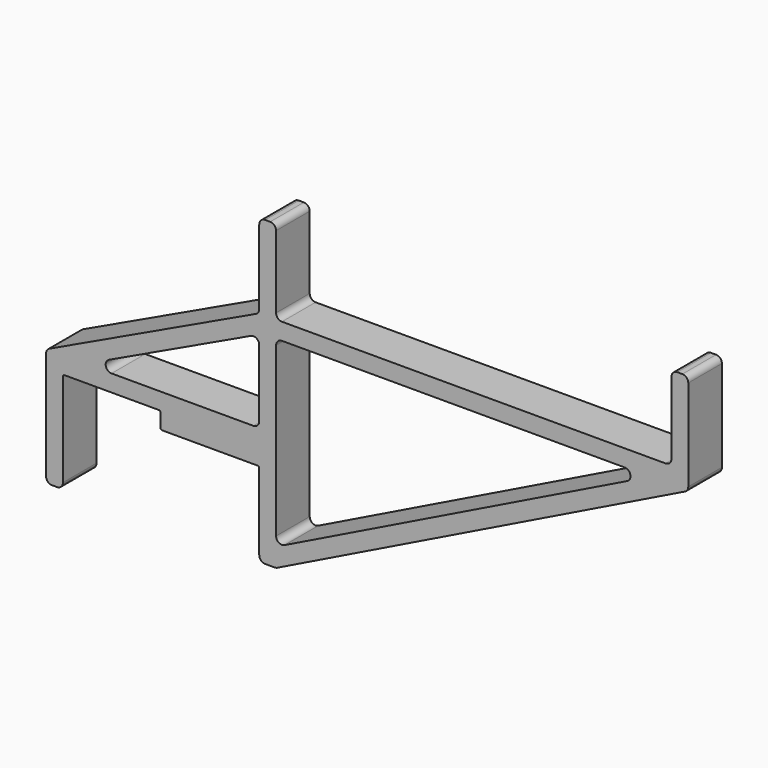
from build123d import *

# Parameters (mm, degrees)
F0_W     = 14.9098
F0_H     = 2.54
F0_W_2   = 2.54
F0_H_2   = 12.7
F1_DEPTH = 6.35
F2_R     = 0.889
F3_R     = 0.254


# Not quite as in the source:
# - a feature names something its author has since deleted; it is built from what else it names


with BuildPart() as f1:
    # F0 (on Front) → F1 (new body)
    with BuildSketch(Plane.XZ):
        Polygon((32.1818, 20.32), (32.1818, 17.78), (34.7218, 17.78), (34.7218, 30.48), (34.7218, 33.02), (32.1818, 33.02), (32.1818, 30.2095859146), align=None)
        Polygon((34.7218, 17.78), (32.1818, 17.78), (32.1818, 15.24), (32.1818, 12.7), (32.1818, 0), (34.7218, 0), (34.7218, 2.8283102922), (34.7218, 13.97), align=None)
        Polygon((0, 17.78), (2.54, 17.78), (5.9346577437, 17.78), (32.1818, 30.2095859146), (32.1818, 33.02), align=None)
        Polygon((5.9346577437, 17.78), (2.54, 17.78), (2.54, 15.24), (17.272, 15.24), (32.1818, 15.24), (32.1818, 17.78), align=None)
        with Locations((24.7269, 13.97)):
            Rectangle(F0_W, F0_H)
        Polygon((2.54, 15.24), (2.54, 17.78), (0, 17.78), (0, 0), (2.54, 0), align=None)
        Polygon((91.1773331535, 30.48), (34.7218, 2.8283102922), (34.7218, 0), (96.9518, 30.48), align=None)
        Polygon((94.4118, 33.02), (34.7218, 33.02), (34.7218, 30.48), (91.1773331535, 30.48), (96.9518, 30.48), (96.9518, 33.02), align=None)
        with Locations((95.6818, 39.37)):
            Rectangle(F0_W_2, F0_H_2)
        with Locations((33.4518, 39.37)):
            Rectangle(F0_W_2, F0_H_2)
    extrude(amount=F1_DEPTH)

    # F2
    f2_edges = [f1.edges().sort_by_distance(p)[0] for p in [
        (0, -3.175, 0),
        (2.54, -3.175, 0),
        (32.1818, -3.175, 0),
        (34.7218, -3.175, 0),
        (32.1818, -3.175, 33.02),
        (0, -3.175, 17.78),
        (32.1818, -3.175, 17.78),
        (32.1818, -3.175, 30.209586),
        (5.934658, -3.175, 17.78),
        (34.7218, -3.175, 2.82831),
        (34.7218, -3.175, 30.48),
        (91.177333, -3.175, 30.48),
        (96.9518, -3.175, 30.48),
        (96.9518, -3.175, 45.72),
        (94.4118, -3.175, 45.72),
        (94.4118, -3.175, 33.02),
        (32.1818, -3.175, 45.72),
        (34.7218, -3.175, 45.72),
        (34.7218, -3.175, 33.02),
    ]]
    fillet(f2_edges, radius=F2_R)

    # F3
    f3_edges = [f1.edges().sort_by_distance(p)[0] for p in [
        (2.54, -3.175, 15.24),
        (17.272, -3.175, 15.24),
        (17.272, -3.175, 12.7),
        (32.1818, -3.175, 12.7),
    ]]
    fillet(f3_edges, radius=F3_R)


solid = f1.part
